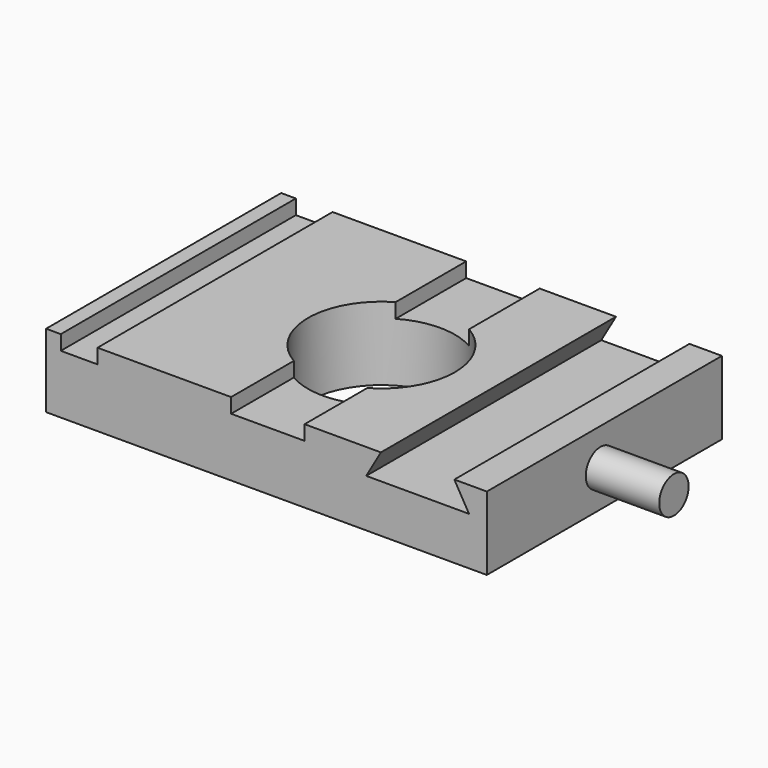
from build123d import *

# Parameters (mm, degrees)
F0_W     = 76.2
F0_H     = 50.8
F0_R     = 12.7
F1_DEPTH = 12.7
F2_W     = 6.35
F2_H     = 50.8
F3_DEPTH = 2.54
F5_DEPTH = 58
F6_R     = 3.175
F7_DEPTH = 12.7


# Not quite as in the source:
# - a feature names something its author has since deleted; it is built from what else it names


with BuildPart() as f1:
    # F0 (on Top) → F1 (new body)
    with BuildSketch(Plane.XY):
        with Locations((-0.2381126344, 0.8489250481)):
            Rectangle(F0_W, F0_H)
        Circle(F0_R, mode=Mode.SUBTRACT)
    extrude(amount=F1_DEPTH)

    # F2 (on face) → F3 (cut)
    with BuildSketch(Plane.XY.offset(12.7)):
        with BuildLine():
            Line((6.35, 26.2489250481), (-6.35, 26.2489250481))
            Line((-6.35, 26.2489250481), (-6.35, 10.9985226281))
            ThreePointArc((-6.35, 10.9985226281), (0, 12.7), (6.35, 10.9985226281))
            Line((6.35, 10.9985226281), (6.35, 26.2489250481))
        make_face()
        with BuildLine():
            ThreePointArc((6.35, -10.9985226281), (0, -12.7), (-6.35, -10.9985226281))
            Line((-6.35, -10.9985226281), (-6.35, -24.5510749519))
            Line((-6.35, -24.5510749519), (6.35, -24.5510749519))
            Line((6.35, -24.5510749519), (6.35, -10.9985226281))
        make_face()
        with Locations((-32.6231126344, 0.8489250481)):
            Rectangle(F2_W, F2_H)
    extrude(amount=-F3_DEPTH, mode=Mode.SUBTRACT)

    # F4 (on face) → F5 (cut)
    with BuildSketch(Plane.XZ.offset(24.5510749519)):
        Polygon((32.2451825857, 12.7), (19.5451825857, 12.7), (17.0051825857, 8.3005909488), (34.7851825857, 8.3005909488), align=None)
    extrude(amount=-F5_DEPTH, mode=Mode.SUBTRACT)

    # F6 (on face) → F7 (join)
    with BuildSketch(Plane.YZ.offset(37.8618873656)):
        with Locations((0, 6.35)):
            Circle(F6_R)
    extrude(amount=F7_DEPTH)


solid = f1.part
